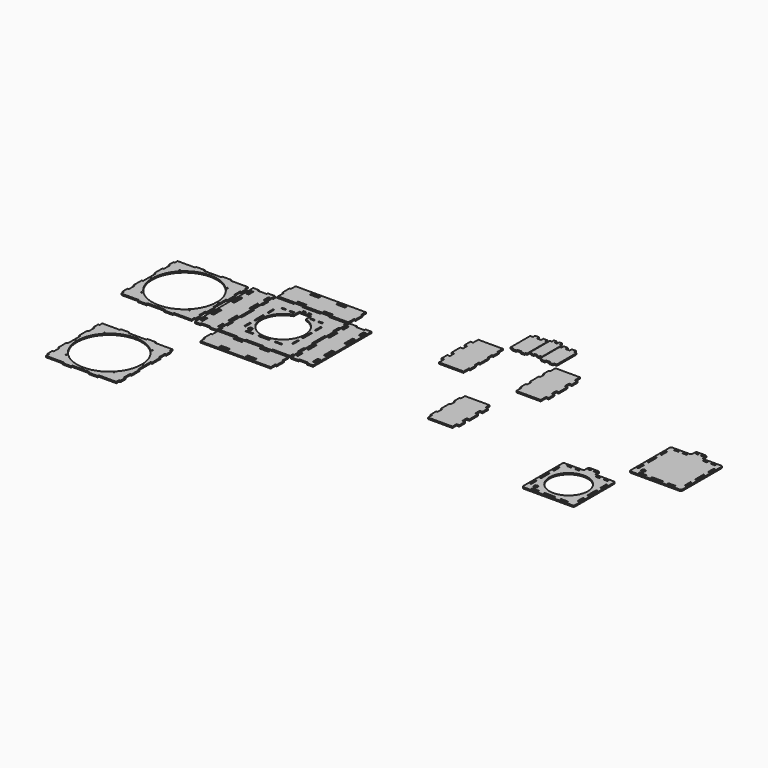
from build123d import *

# Parameters (mm, degrees)
F0_R     = 2
F0_R_2   = 118.6639071569
F1_DEPTH = 5
F0_W     = 32.25
F0_H     = 5
F0_W_2   = 26
F0_R_3   = 7.0999608773
F0_W_3   = 5
F0_H_2   = 26
F0_W_4   = 15
F0_W_5   = 10
F0_H_3   = 22.5386619568
F0_H_4   = 37.4457836151
F0_W_6   = 5.0000161439
F0_W_7   = 40
F0_R_4   = 70


# Not quite as in the source:
# - ends of sketch curves that miss each other by under 0.0002 mm in the source are joined


with BuildPart() as f1:
    # F0 (on Top) → F1 (new body)
    with BuildSketch(Plane.XY):
        Polygon((-1366.6140356064, -884.7837514877), (-1366.6140356064, -897.4375081062), (-1302.1140356064, -897.4375081062), (-1302.1140356064, -902.4375081062), (-1269.8640356064, -902.4375081062), (-1269.8640356064, -897.4375081062), (-1205.3640356064, -897.4375081062), (-1205.3640356064, -902.4375081062), (-1173.1140356064, -902.4375081062), (-1173.1140356064, -897.4375081062), (-1108.6140356064, -897.4375081062), (-1108.6140356064, -884.7837514877), (-1103.6140356064, -884.7837514877), (-1103.6140356064, -862.2450895309), (-1108.6140356064, -862.2450895309), (-1108.6140356064, -834.8589010239), (-1103.6140356064, -834.8589010239), (-1103.6140356064, -797.4131174088), (-1108.6140356064, -797.4131174088), (-1108.6140356064, -739.4618988037), (-1103.6140356064, -739.4618988037), (-1103.6140356064, -702.0161151886), (-1108.6140356064, -702.0161151886), (-1108.6140356064, -674.6299266815), (-1103.6140356064, -674.6299266815), (-1103.6140356064, -652.0912647247), (-1108.6140356064, -652.0912647247), (-1108.6140356064, -639.4375081062), (-1173.1140356064, -639.4375081062), (-1173.1140356064, -634.4375081062), (-1205.3640356064, -634.4375081062), (-1205.3640356064, -639.4375081062), (-1269.8640356064, -639.4375081062), (-1269.8640356064, -634.4375081062), (-1302.1140356064, -634.4375081062), (-1302.1140356064, -639.4375081062), (-1366.6140356064, -639.4375081062), (-1366.6140356064, -652.0912647247), (-1371.6140356064, -652.0912647247), (-1371.6140356064, -674.6299266815), (-1366.6140356064, -674.6299266815), (-1366.6140356064, -702.0161151886), (-1371.6140356064, -702.0161151886), (-1371.6140356064, -739.4618988037), (-1366.6140356064, -739.4618988037), (-1366.6140356064, -797.4131174088), (-1371.6140356064, -797.4131174088), (-1371.6140356064, -834.8589010239), (-1366.6140356064, -834.8589010239), (-1366.6140356064, -862.2450895309), (-1371.6140356064, -862.2450895309), (-1371.6140356064, -884.7837514877), align=None)
        with Locations((-1325.1184997782, -855.9419722781)):
            Circle(F0_R, mode=Mode.SUBTRACT)
        with Locations((-1237.6140356064, -892.1875081062)):
            Circle(F0_R, mode=Mode.SUBTRACT)
        with Locations((-1150.1095714345, -855.9419722781)):
            Circle(F0_R, mode=Mode.SUBTRACT)
        with Locations((-1361.3640356064, -768.4375081062)):
            Circle(F0_R, mode=Mode.SUBTRACT)
        with Locations((-1237.6140356064, -768.4375081062)):
            Circle(F0_R_2, mode=Mode.SUBTRACT)
        with Locations((-1113.8640356064, -768.4375081062)):
            Circle(F0_R, mode=Mode.SUBTRACT)
        with Locations((-1325.1184997782, -680.9330439344)):
            Circle(F0_R, mode=Mode.SUBTRACT)
        with Locations((-1150.1095714345, -680.9330439344)):
            Circle(F0_R, mode=Mode.SUBTRACT)
        with BuildLine():
            ThreePointArc((-1237.6140356064, -646.6875081062), (-1239.0282491688, -643.2732945439), (-1235.6140356064, -644.6875081062))
            ThreePointArc((-1235.6140356064, -644.6875081062), (-1236.199822044, -646.1017216686), (-1237.6140356064, -646.6875081062))
        make_face(mode=Mode.SUBTRACT)
    extrude(amount=F1_DEPTH)


with BuildPart() as f1b:
    # F0 (on Top) → F1, piece 2 (new body)
    with BuildSketch(Plane.XY):
        Polygon((-1293.2458279068, -1321.7081812524), (-1293.2458279068, -1334.3619378709), (-1228.7458279068, -1334.3619378709), (-1228.7458279068, -1339.3619378709), (-1196.4958279068, -1339.3619378709), (-1196.4958279068, -1334.3619378709), (-1131.9958279068, -1334.3619378709), (-1131.9958279068, -1339.3619378709), (-1099.7458279068, -1339.3619378709), (-1099.7458279068, -1334.3619378709), (-1035.2458279068, -1334.3619378709), (-1035.2458279068, -1321.7081812524), (-1030.2458279068, -1321.7081812524), (-1030.2458279068, -1299.1695192956), (-1035.2458279068, -1299.1695192956), (-1035.2458279068, -1271.7833307885), (-1030.2458279068, -1271.7833307885), (-1030.2458279068, -1234.3375471734), (-1035.2458279068, -1234.3375471734), (-1035.2458279068, -1176.3863285683), (-1030.2458279068, -1176.3863285683), (-1030.2458279068, -1138.9405449532), (-1035.2458279068, -1138.9405449532), (-1035.2458279068, -1111.5543564461), (-1030.2458279068, -1111.5543564461), (-1030.2458279068, -1089.0156944894), (-1035.2458279068, -1089.0156944894), (-1035.2458279068, -1076.3619378709), (-1099.7458279068, -1076.3619378709), (-1099.7458279068, -1071.3619378709), (-1131.9958279068, -1071.3619378709), (-1131.9958279068, -1076.3619378709), (-1196.4958279068, -1076.3619378709), (-1196.4958279068, -1071.3619378709), (-1228.7458279068, -1071.3619378709), (-1228.7458279068, -1076.3619378709), (-1293.2458279068, -1076.3619378709), (-1293.2458279068, -1089.0156944894), (-1298.2458279068, -1089.0156944894), (-1298.2458279068, -1111.5543564461), (-1293.2458279068, -1111.5543564461), (-1293.2458279068, -1138.9405449532), (-1298.2458279068, -1138.9405449532), (-1298.2458279068, -1176.3863285683), (-1293.2458279068, -1176.3863285683), (-1293.2458279068, -1234.3375471734), (-1298.2458279068, -1234.3375471734), (-1298.2458279068, -1271.7833307885), (-1293.2458279068, -1271.7833307885), (-1293.2458279068, -1299.1695192956), (-1298.2458279068, -1299.1695192956), (-1298.2458279068, -1321.7081812524), align=None)
        with Locations((-1251.7502920787, -1292.8664020427)):
            Circle(F0_R, mode=Mode.SUBTRACT)
        with Locations((-1164.2458279068, -1329.1119378709)):
            Circle(F0_R, mode=Mode.SUBTRACT)
        with Locations((-1287.9958279068, -1205.3619378709)):
            Circle(F0_R, mode=Mode.SUBTRACT)
        with Locations((-1164.2458279068, -1205.3619378709)):
            Circle(F0_R_2, mode=Mode.SUBTRACT)
        with Locations((-1076.741363735, -1292.8664020427)):
            Circle(F0_R, mode=Mode.SUBTRACT)
        with Locations((-1040.4958279068, -1205.3619378709)):
            Circle(F0_R, mode=Mode.SUBTRACT)
        with Locations((-1251.7502920787, -1117.857473699)):
            Circle(F0_R, mode=Mode.SUBTRACT)
        with BuildLine():
            ThreePointArc((-1164.2458279068, -1083.6119378709), (-1165.6600414692, -1080.1977243085), (-1162.2458279068, -1081.6119378709))
            ThreePointArc((-1162.2458279068, -1081.6119378709), (-1162.8316143445, -1083.0261514332), (-1164.2458279068, -1083.6119378709))
        make_face(mode=Mode.SUBTRACT)
        with Locations((-1076.741363735, -1117.857473699)):
            Circle(F0_R, mode=Mode.SUBTRACT)
    extrude(amount=F1_DEPTH)


with BuildPart() as f1c:
    # F0 (on Top) → F1, piece 3 (new body)
    with BuildSketch(Plane.XY):
        Polygon((-1004.6137704086, -965.3843326569), (-1004.6137704086, -971.6343326569), (-1004.6137704086, -981.6343326569), (-1004.6137704086, -986.6343326569), (-746.6137704086, -986.6343326569), (-746.6137704086, -981.6343326569), (-746.6137704086, -965.3843326569), (-741.6137704086, -965.3843326569), (-741.6137704086, -932.8843326569), (-746.6137704086, -932.8843326569), (-746.6137704086, -911.6343326569), (-746.6137704086, -906.6343326569), (-1004.6137704086, -906.6343326569), (-1004.6137704086, -911.6343326569), (-1004.6137704086, -932.8843326569), (-1009.6137704086, -932.8843326569), (-1009.6137704086, -965.3843326569), align=None)
        Polygon((-907.8637704086, -971.6343326569), (-907.8637704086, -976.6343326569), (-907.8637704086, -981.6343326569), (-940.1137704086, -981.6343326569), (-940.1137704086, -976.6343326569), (-940.1137704086, -971.6343326569), align=None, mode=Mode.SUBTRACT)
        with Locations((-923.9887704086, -914.1343326569)):
            Rectangle(F0_W, F0_H, mode=Mode.SUBTRACT)
        Polygon((-811.1137704086, -971.6343326569), (-811.1137704086, -976.6343326569), (-811.1137704086, -981.6343326569), (-843.3637704086, -981.6343326569), (-843.3637704086, -976.6343326569), (-843.3637704086, -971.6343326569), align=None, mode=Mode.SUBTRACT)
        with Locations((-827.2387704086, -914.1343326569)):
            Rectangle(F0_W, F0_H, mode=Mode.SUBTRACT)
    extrude(amount=F1_DEPTH)


with BuildPart() as f1d:
    # F0 (on Top) → F1, piece 4 (new body)
    with BuildSketch(Plane.XY):
        Polygon((-907.8637704086, -634.4375081062), (-940.1137704086, -634.4375081062), (-940.1137704086, -639.4375081062), (-1004.6137704086, -639.4375081062), (-1004.6137704086, -652.0912647247), (-1009.6137704086, -652.0912647247), (-1009.6137704086, -674.6299266815), (-1004.6137704086, -674.6299266815), (-1004.6137704086, -678.4375081062), (-1004.6137704086, -702.0161151886), (-1009.6137704086, -702.0161151886), (-1009.6137704086, -718.4375081062), (-1009.6137704086, -739.4618988037), (-1004.6137704086, -739.4618988037), (-1004.6137704086, -748.4375081062), (-1004.6137704086, -788.3375081062), (-1004.6137704086, -788.4375081062), (-1004.6137704086, -797.4131174088), (-1009.6137704086, -797.4131174088), (-1009.6137704086, -818.4375081062), (-1009.6137704086, -834.8589010239), (-1004.6137704086, -834.8589010239), (-1004.6137704086, -858.4375081062), (-1004.6137704086, -862.2450895309), (-1009.6137704086, -862.2450895309), (-1009.6137704086, -884.7837514877), (-1004.6137704086, -884.7837514877), (-1004.6137704086, -897.4375081062), (-940.1137704086, -897.4375081062), (-940.1137704086, -902.4375081062), (-907.8637704086, -902.4375081062), (-907.8637704086, -897.4375081062), (-843.3637704086, -897.4375081062), (-843.3637704086, -902.4375081062), (-811.1137704086, -902.4375081062), (-811.1137704086, -897.4375081062), (-746.6137704086, -897.4375081062), (-746.6137704086, -884.7837514877), (-741.6137704086, -884.7837514877), (-741.6137704086, -862.2450895309), (-746.6137704086, -862.2450895309), (-746.6137704086, -858.4375081062), (-746.6137704086, -834.8589010239), (-741.6137704086, -834.8589010239), (-741.6137704086, -818.4375081062), (-741.6137704086, -797.4131174088), (-746.6137704086, -797.4131174088), (-746.6137704086, -788.3375081062), (-746.6137704086, -748.4375081062), (-746.6137704086, -739.4618988037), (-741.6137704086, -739.4618988037), (-741.6137704086, -718.4375081062), (-741.6137704086, -702.0161151886), (-746.6137704086, -702.0161151886), (-746.6137704086, -678.4375081062), (-746.6137704086, -674.6299266815), (-741.6137704086, -674.6299266815), (-741.6137704086, -652.0912647247), (-746.6137704086, -652.0912647247), (-746.6137704086, -639.4375081062), (-811.1137704086, -639.4375081062), (-811.1137704086, -634.4375081062), (-843.3637704086, -634.4375081062), (-843.3637704086, -639.4375081062), (-907.8637704086, -639.4375081062), align=None)
        with Locations((-928.6137704086, -855.9375081062)):
            Rectangle(F0_W_2, F0_H, mode=Mode.SUBTRACT)
        Polygon((-895.6137704086, -858.4375081062), (-895.6137704086, -853.4375081062), (-855.6137704086, -853.4375081062), (-855.6137704086, -858.4375081062), (-875.6137704086, -858.4375081062), align=None, mode=Mode.SUBTRACT)
        with Locations((-940.6262636185, -837.5561237335)):
            Circle(F0_R_3, mode=Mode.SUBTRACT)
        with Locations((-963.1137704086, -821.4375081062)):
            Rectangle(F0_W_3, F0_H_2, mode=Mode.SUBTRACT)
        Polygon((-960.6137704086, -748.4375081062), (-960.6137704086, -768.4375081062), (-960.6137704086, -788.4375081062), (-965.6137704086, -788.4375081062), (-965.6137704086, -748.4375081062), align=None, mode=Mode.SUBTRACT)
        with BuildLine():
            ThreePointArc((-955.6137704086, -768.4375081062), (-939.4886480993, -720.2711297911), (-897.6137704086, -691.5219700141))
            Line((-897.6137704086, -691.5219700141), (-897.6137704086, -666.4375081062))
            Line((-897.6137704086, -666.4375081062), (-875.6137704086, -666.4375081062))
            Line((-875.6137704086, -666.4375081062), (-870.7256383133, -666.4375081062))
            Line((-870.7256383133, -666.4375081062), (-853.6137704086, -666.4375081062))
            Line((-853.6137704086, -666.4375081062), (-853.6137704086, -691.5219700141))
            ThreePointArc((-853.6137704086, -691.5219700141), (-811.7388927179, -720.2711297911), (-795.6137704086, -768.4375081062))
            ThreePointArc((-795.6137704086, -768.4375081062), (-819.0452279137, -825.0060506012), (-875.6137704086, -848.4375081062))
            ThreePointArc((-875.6137704086, -848.4375081062), (-932.1823129036, -825.0060506012), (-955.6137704086, -768.4375081062))
        make_face(mode=Mode.SUBTRACT)
        with Locations((-963.1137704086, -715.4375081062)):
            Rectangle(F0_W_3, F0_H_2, mode=Mode.SUBTRACT)
        with Locations((-822.6137704086, -855.9375081062)):
            Rectangle(F0_W_2, F0_H, mode=Mode.SUBTRACT)
        with Locations((-788.1137704086, -821.4375081062)):
            Rectangle(F0_W_3, F0_H_2, mode=Mode.SUBTRACT)
        Polygon((-790.6137704086, -768.4375081062), (-790.6137704086, -748.4375081062), (-785.6137704086, -748.4375081062), (-785.6137704086, -768.4375081062), (-785.6137704086, -788.4375081062), (-790.6137704086, -788.4375081062), align=None, mode=Mode.SUBTRACT)
        with Locations((-788.1137704086, -715.4375081062)):
            Rectangle(F0_W_3, F0_H_2, mode=Mode.SUBTRACT)
        with Locations((-943.1137704086, -680.9375081062)):
            Rectangle(F0_W_4, F0_H, mode=Mode.SUBTRACT)
        with Locations((-913.1137704086, -680.9375081062)):
            Rectangle(F0_W_4, F0_H, mode=Mode.SUBTRACT)
        with Locations((-885.6137704086, -658.9375081062)):
            Rectangle(F0_W_5, F0_H, mode=Mode.SUBTRACT)
        with Locations((-838.1137704086, -680.9375081062)):
            Rectangle(F0_W_4, F0_H, mode=Mode.SUBTRACT)
        with Locations((-808.1137704086, -680.9375081062)):
            Rectangle(F0_W_4, F0_H, mode=Mode.SUBTRACT)
        with Locations((-865.6137704086, -658.9375081062)):
            Rectangle(F0_W_5, F0_H, mode=Mode.SUBTRACT)
    extrude(amount=F1_DEPTH)


with BuildPart() as f1e:
    # F0 (on Top) → F1, piece 5 (new body)
    with BuildSketch(Plane.XY):
        Polygon((-679.8637704086, -634.4375081062), (-679.8637704086, -639.5375081062), (-696.1137704086, -639.5375081062), (-712.3637704086, -639.5375081062), (-712.3637704086, -634.4375081062), (-728.6137704086, -634.4375081062), (-733.6137704086, -634.4375081062), (-738.6137704086, -634.4375081062), (-738.6137704086, -678.4375081062), (-738.6137704086, -858.4375081062), (-738.6137704086, -902.4375081062), (-733.6137704086, -902.4375081062), (-728.6137704086, -902.4375081062), (-712.3637704086, -902.4375081062), (-712.3637704086, -897.4375081062), (-679.8637704086, -897.4375081062), (-679.8637704086, -902.4375081062), (-663.6137704086, -902.4375081062), (-658.6137704086, -902.4375081062), (-658.6137704086, -634.4375081062), (-663.6137704086, -634.4375081062), align=None)
        with Locations((-731.1137704086, -873.5144205093)):
            Rectangle(F0_W_3, F0_H_3, mode=Mode.SUBTRACT)
        Polygon((-673.6137704086, -862.2450895309), (-668.6137704086, -862.2450895309), (-663.6137704086, -862.2450895309), (-663.6137704086, -884.7837514877), (-668.6137704086, -884.7837514877), (-673.6137704086, -884.7837514877), align=None, mode=Mode.SUBTRACT)
        with Locations((-731.1137704086, -816.1360092163)):
            Rectangle(F0_W_3, F0_H_4, mode=Mode.SUBTRACT)
        Polygon((-673.6137704086, -797.4131174088), (-668.6137704086, -797.4131174088), (-663.6137704086, -797.4131174088), (-663.6137704086, -834.8589010239), (-668.6137704086, -834.8589010239), (-673.6137704086, -834.8589010239), align=None, mode=Mode.SUBTRACT)
        Polygon((-733.6137704086, -702.0161151886), (-728.6137704086, -702.0161151886), (-728.6137704086, -739.4618988037), (-733.6137704086, -739.4618988037), (-733.6137704086, -718.4375081062), align=None, mode=Mode.SUBTRACT)
        Polygon((-668.6137704086, -739.4618988037), (-673.6137704086, -739.4618988037), (-673.6137704086, -702.0161151886), (-668.6137704086, -702.0161151886), (-663.6137704086, -702.0161151886), (-663.6137704086, -739.4618988037), align=None, mode=Mode.SUBTRACT)
        with Locations((-731.1137704086, -663.3605957031)):
            Rectangle(F0_W_3, F0_H_3, mode=Mode.SUBTRACT)
        Polygon((-673.6137704086, -652.0912647247), (-668.6137704086, -652.0912647247), (-663.6137704086, -652.0912647247), (-663.6137704086, -674.6299266815), (-668.6137704086, -674.6299266815), (-673.6137704086, -674.6299266815), align=None, mode=Mode.SUBTRACT)
    extrude(amount=F1_DEPTH)


with BuildPart() as f1f:
    # F0 (on Top) → F1, piece 6 (new body)
    with BuildSketch(Plane.XY):
        Polygon((-1017.6137704086, -634.4375081062), (-1022.6137704086, -634.4375081062), (-1038.8637704086, -634.4375081062), (-1038.8637704086, -639.5375081062), (-1055.1137704086, -639.5375081062), (-1071.3637704086, -639.5375081062), (-1071.3637704086, -634.4375081062), (-1087.6137704086, -634.4375081062), (-1092.6137704086, -634.4375081062), (-1092.6137704086, -902.4375081062), (-1087.6137704086, -902.4375081062), (-1071.3637704086, -902.4375081062), (-1071.3637704086, -897.4375081062), (-1038.8637704086, -897.4375081062), (-1038.8637704086, -902.4375081062), (-1022.6137704086, -902.4375081062), (-1017.6137704086, -902.4375081062), (-1012.6137704086, -902.4375081062), (-1012.6137704086, -858.4375081062), (-1012.6137704086, -678.4375081062), (-1012.6137704086, -634.4375081062), align=None)
        Polygon((-1082.6137704086, -884.7837514877), (-1087.6137704086, -884.7837514877), (-1087.6137704086, -862.2450895309), (-1082.6137704086, -862.2450895309), (-1077.6137704086, -862.2450895309), (-1077.6137704086, -884.7837514877), align=None, mode=Mode.SUBTRACT)
        with Locations((-1020.1137704086, -873.5144205093)):
            Rectangle(F0_W_3, F0_H_3, mode=Mode.SUBTRACT)
        Polygon((-1082.6137704086, -834.8589010239), (-1087.6137704086, -834.8589010239), (-1087.6137704086, -797.4131174088), (-1082.6137704086, -797.4131174088), (-1077.6137704086, -797.4131174088), (-1077.6137704086, -834.8589010239), align=None, mode=Mode.SUBTRACT)
        with Locations((-1020.1137704086, -816.1360092163)):
            Rectangle(F0_W_3, F0_H_4, mode=Mode.SUBTRACT)
        Polygon((-1087.6137704086, -739.4618988037), (-1087.6137704086, -702.0161151886), (-1082.6137704086, -702.0161151886), (-1077.6137704086, -702.0161151886), (-1077.6137704086, -739.4618988037), (-1082.6137704086, -739.4618988037), align=None, mode=Mode.SUBTRACT)
        Polygon((-1017.6137704086, -739.4618988037), (-1022.6137704086, -739.4618988037), (-1022.6137704086, -702.0161151886), (-1017.6137704086, -702.0161151886), (-1017.6137704086, -718.4375081062), align=None, mode=Mode.SUBTRACT)
        Polygon((-1087.6137704086, -674.6299266815), (-1087.6137704086, -652.0912647247), (-1082.6137704086, -652.0912647247), (-1077.6137704086, -652.0912647247), (-1077.6137704086, -674.6299266815), (-1082.6137704086, -674.6299266815), align=None, mode=Mode.SUBTRACT)
        with Locations((-1020.1137704086, -663.3605957031)):
            Rectangle(F0_W_3, F0_H_3, mode=Mode.SUBTRACT)
    extrude(amount=F1_DEPTH)


with BuildPart() as f1g:
    # F0 (on Top) → F1, piece 7 (new body)
    with BuildSketch(Plane.XY):
        Polygon((-1004.6137704086, -620.2406835556), (-1004.6137704086, -625.2406835556), (-1004.6137704086, -630.2406835556), (-940.1137704086, -630.2406835556), (-746.6137704086, -630.2406835556), (-746.6137704086, -625.2406835556), (-746.6137704086, -603.9906835556), (-741.6137704086, -603.9906835556), (-741.6137704086, -571.4906835556), (-746.6137704086, -571.4906835556), (-746.6137704086, -555.2406835556), (-746.6137704086, -550.2406835556), (-1004.6137704086, -550.2406835556), (-1004.6137704086, -555.2406835556), (-1004.6137704086, -565.2406835556), (-1004.6137704086, -571.4906835556), (-1009.6137704086, -571.4906835556), (-1009.6137704086, -603.9906835556), (-1004.6137704086, -603.9906835556), align=None)
        with Locations((-923.9887704086, -622.7406835556)):
            Rectangle(F0_W, F0_H, mode=Mode.SUBTRACT)
        Polygon((-940.1137704086, -565.2406835556), (-940.1137704086, -560.2406835556), (-940.1137704086, -555.2406835556), (-907.8637704086, -555.2406835556), (-907.8637704086, -560.2406835556), (-907.8637704086, -565.2406835556), align=None, mode=Mode.SUBTRACT)
        with Locations((-827.2387704086, -622.7406835556)):
            Rectangle(F0_W, F0_H, mode=Mode.SUBTRACT)
        Polygon((-811.1137704086, -555.2406835556), (-811.1137704086, -560.2406835556), (-811.1137704086, -565.2406835556), (-843.3637704086, -565.2406835556), (-843.3637704086, -560.2406835556), (-843.3637704086, -555.2406835556), align=None, mode=Mode.SUBTRACT)
    extrude(amount=F1_DEPTH)


with BuildPart() as f1h:
    # F0 (on Top) → F1, piece 8 (new body)
    with BuildSketch(Plane.XY):
        Polygon((-298.4449183991, -662.1296386563), (-298.1309330463, -662.1296386563), (-298.1309330463, -638.1296386563), (-293.1309330463, -638.1296386563), (-293.1309330463, -612.1296386563), (-298.1309330463, -612.1296386563), (-298.1309330463, -592.1296386563), (-293.1309330463, -592.1296386563), (-293.1309330463, -552.1665781096), (-298.1309330463, -552.1665781096), (-298.1309330463, -532.1665781096), (-293.1309330463, -532.1665781096), (-293.1309330463, -506.1665781096), (-298.1309330463, -506.1296386563), (-298.1309330463, -482.1296386563), (-383.1309330463, -482.1296386563), (-388.1309330463, -482.1296386563), (-388.1309330463, -492.7178739505), (-388.1309330463, -506.1296386563), (-398.1309330463, -506.1296386563), (-398.1309330463, -532.1665781096), (-388.1309330463, -532.1665781096), (-388.1309330463, -552.1665781096), (-398.1309330463, -552.1665781096), (-398.1309330463, -592.1296386563), (-388.1309330463, -592.1296386563), (-388.1309330463, -612.1296386563), (-398.1309330463, -612.1296386563), (-398.1309330463, -638.1296386563), (-388.1309330463, -638.1296386563), (-388.1309330463, -651.5783428154), (-388.1309330463, -662.1296386563), align=None)
    extrude(amount=F1_DEPTH)


with BuildPart() as f1i:
    # F0 (on Top) → F1, piece 9 (new body)
    with BuildSketch(Plane.XY):
        Polygon((-286.3878677518, -460.9915268421), (-284.3879467788, -460.9915268421), (-276.3878677518, -460.9915268421), (-276.3878677518, -465.9915268421), (-271.3878677518, -465.9915268421), (-261.3878677518, -465.9915268421), (-261.3878677518, -460.9915268421), (-256.9990215546, -460.9915268421), (-246.3878677518, -460.9915268421), (-246.3878677518, -465.9915268421), (-241.3878677518, -465.9915268421), (-231.3878677518, -465.9915268421), (-231.3878677518, -460.9915268421), (-225.3675460815, -461.0270857811), (-225.3675460815, -371.0271845648), (-231.3878677518, -371.0271845648), (-231.3878677518, -361.0270857811), (-241.3878677518, -361.0270857811), (-246.3878677518, -361.0270857811), (-246.3878677518, -371.0271852235), (-256.4324156498, -371.0271852235), (-261.3878677518, -371.0271852235), (-261.3878677518, -361.0270857811), (-276.3878677518, -361.0270857811), (-276.3878677518, -371.0271852235), (-286.3878677518, -371.0271852235), align=None)
    extrude(amount=F1_DEPTH)


with BuildPart() as f1j:
    # F0 (on Top) → F1, piece 10 (new body)
    with BuildSketch(Plane.XY):
        Polygon((-216.3878677518, -359.7890693303), (-223.3878677518, -359.7890693303), (-223.3878677518, -449.7890693303), (-216.3878677518, -449.7890693303), (-216.3878677518, -454.7890693303), (-206.3878677518, -454.7890693303), (-206.3878677518, -449.7890693303), (-201.4541815716, -449.7890693303), (-201.3215539319, -449.7890693303), (-196.3878677518, -449.7890693303), (-196.3878677518, -454.7890693303), (-186.3878677518, -454.7890693303), (-186.3878677518, -449.7890693303), (-179.3878677518, -449.7890693303), (-179.3878677518, -359.7890693303), (-186.3878677518, -359.7890693303), (-186.3878677518, -354.7890693303), (-186.3878677518, -349.7890693303), (-196.3878677518, -349.7890693303), (-196.3878677518, -354.7890693303), (-196.3878677518, -359.7890693303), (-201.3878677518, -359.7890693303), (-206.3878677518, -359.7890693303), (-206.3878677518, -354.7890693303), (-206.3878677518, -349.7890693303), (-216.3878677518, -349.7890693303), (-216.3878677518, -354.7890693303), align=None)
    extrude(amount=F1_DEPTH)


with BuildPart() as f1k:
    # F0 (on Top) → F1, piece 11 (new body)
    with BuildSketch(Plane.XY):
        Polygon((-177.408189422, -371.0271845648), (-177.408189422, -461.0270857811), (-171.3878677518, -460.9915268421), (-171.3878677518, -465.9915268421), (-161.3878677518, -465.9915268421), (-156.3878677518, -465.9915268421), (-156.3878677518, -460.9915268421), (-145.7767139489, -460.9915268421), (-141.3878677518, -460.9915268421), (-141.3878677518, -465.9915268421), (-131.3878677518, -465.9915268421), (-126.3878677518, -465.9915268421), (-126.3878677518, -460.9915268421), (-118.3877887248, -460.9915268421), (-116.3878677518, -460.9915268421), (-116.3878677518, -371.0271852235), (-126.3878677518, -371.0271852235), (-126.3878677518, -361.0270857811), (-141.3878677518, -361.0270857811), (-141.3878677518, -371.0271852235), (-146.3433198538, -371.0271852235), (-156.3878677518, -371.0271852235), (-156.3878677518, -361.0270857811), (-161.3878677518, -361.0270857811), (-171.3878677518, -361.0270857811), (-171.3878677518, -371.0271845648), align=None)
    extrude(amount=F1_DEPTH)


with BuildPart() as f1l:
    # F0 (on Top) → F1, piece 12 (new body)
    with BuildSketch(Plane.XY):
        Polygon((-104.6448024572, -482.1296386563), (-104.6448024572, -506.1296386563), (-109.6448024572, -506.1665781096), (-109.6448024572, -532.1665781096), (-104.6448024572, -532.1665781096), (-104.6448024572, -552.1665781096), (-109.6448024572, -552.1665781096), (-109.6448024572, -592.1296386563), (-104.6448024572, -592.1296386563), (-104.6448024572, -612.1296386563), (-109.6448024572, -612.1296386563), (-109.6448024572, -638.1296386563), (-104.6448024572, -638.1296386563), (-104.6448024572, -662.1296386563), (-104.3308171044, -662.1296386563), (-14.6448024572, -662.1296386563), (-14.6448024572, -651.5783428154), (-14.6448024572, -638.1296386563), (-4.6448024572, -638.1296386563), (-4.6448024572, -612.1296386563), (-14.6448024572, -612.1296386563), (-14.6448024572, -592.1296386563), (-4.6448024572, -592.1296386563), (-4.6448024572, -552.1665781096), (-14.6448024572, -552.1665781096), (-14.6448024572, -532.1665781096), (-4.6448024572, -532.1665781096), (-4.6448024572, -506.1296386563), (-14.6448024572, -506.1296386563), (-14.6448024572, -492.7178739505), (-14.6448024572, -482.1296386563), (-19.6448024572, -482.1296386563), align=None)
    extrude(amount=F1_DEPTH)


with BuildPart() as f1m:
    # F0 (on Top) → F1, piece 13 (new body)
    with BuildSketch(Plane.XY):
        Polygon((-199.1916574645, -780.1817527555), (-199.1916574645, -798.1817527555), (-204.1916574645, -798.2186922088), (-204.1916574645, -824.2186922088), (-199.1916574645, -824.2186922088), (-199.1916574645, -844.2186922088), (-204.1916574645, -844.2186922088), (-204.1916574645, -884.1817527555), (-199.1916574645, -884.1817527555), (-199.1916574645, -904.1817527555), (-204.1916574645, -904.1817527555), (-204.1916574645, -930.1817527555), (-199.1916574645, -930.1817527555), (-199.1916574645, -948.2556316621), (-199.1916574645, -949.2556316621), (-109.1916574645, -949.2556316621), (-109.1916574645, -938.6673963679), (-109.1916574645, -930.1817527555), (-99.1916574645, -930.1817527555), (-99.1916574645, -904.1817527555), (-109.1916574645, -904.1817527555), (-109.1916574645, -884.1817527555), (-99.1916574645, -884.1817527555), (-99.1916574645, -844.2186922088), (-109.1916574645, -844.2186922088), (-109.1916574645, -824.2186922088), (-99.1916574645, -824.2186922088), (-99.1916574645, -798.1817527555), (-109.1916574645, -798.1817527555), (-109.1916574645, -789.7699880497), (-109.1916574645, -779.1817527555), (-199.1916574645, -779.1817527555), align=None)
    extrude(amount=F1_DEPTH)


with BuildPart() as f1n:
    # F0 (on Top) → F1, piece 14 (new body)
    with BuildSketch(Plane.XY):
        with BuildLine():
            Line((464.3994565253, -847.4577746544), (488.3994726692, -847.4577746544))
            Line((488.3994726692, -847.4577746544), (644.3994565253, -847.4577746544))
            ThreePointArc((644.3994565253, -847.4577746544), (647.9349904312, -845.9933085603), (649.3994565253, -842.4577746544))
            Line((649.3994565253, -842.4577746544), (649.3994565253, -662.4577746544))
            ThreePointArc((649.3994565253, -662.4577746544), (647.9349904312, -658.9222407484), (644.3994565253, -657.4577746544))
            Line((644.3994565253, -657.4577746544), (579.3994565253, -657.4577746544))
            ThreePointArc((579.3994565253, -657.4577746544), (575.8639226194, -655.9933085603), (574.3994565253, -652.4577746544))
            Line((574.3994565253, -652.4577746544), (574.3994565253, -650.476244381))
            Line((574.3994565253, -650.476244381), (574.3994565253, -645.476244381))
            Line((574.3994565253, -645.476244381), (574.3994565253, -640.476244381))
            ThreePointArc((574.3994565253, -640.476244381), (572.9349904312, -636.9406895606), (569.3994565253, -635.4762234665))
            Line((569.3994565253, -635.4762234665), (539.3994565253, -635.4762234665))
            ThreePointArc((539.3994565253, -635.4762234665), (535.8639226194, -636.9406895606), (534.3994565253, -640.4762234665))
            Line((534.3994565253, -640.4762234665), (534.3994565253, -652.4577746544))
            ThreePointArc((534.3994565253, -652.4577746544), (532.9349904312, -655.9933085603), (529.3994565253, -657.4577746544))
            Line((529.3994565253, -657.4577746544), (464.3994565253, -657.4577746544))
            ThreePointArc((464.3994565253, -657.4577746544), (460.8639226194, -658.9222407484), (459.3994565253, -662.4577746544))
            Line((459.3994565253, -662.4577746544), (459.3994565253, -752.4947141076))
            Line((459.3994565253, -752.4947141076), (459.3994565253, -842.4577746544))
            ThreePointArc((459.3994565253, -842.4577746544), (460.8639226194, -845.9933085603), (464.3994565253, -847.4577746544))
        make_face()
        with Locations((501.3994726692, -839.9577746544)):
            Rectangle(F0_W_2, F0_H, mode=Mode.SUBTRACT)
        with Locations((489.3869633155, -821.5763902817)):
            Circle(F0_R_3, mode=Mode.SUBTRACT)
        with Locations((466.8994645973, -805.4577746544)):
            Rectangle(F0_W_6, F0_H_2, mode=Mode.SUBTRACT)
        with Locations((554.3994726692, -839.9577746544)):
            Rectangle(F0_W_7, F0_H, mode=Mode.SUBTRACT)
        with Locations((607.3994726692, -839.9577746544)):
            Rectangle(F0_W_2, F0_H, mode=Mode.SUBTRACT)
        with Locations((641.8994484533, -805.4577746544)):
            Rectangle(F0_W_6, F0_H_2, mode=Mode.SUBTRACT)
        Polygon((469.3994565253, -752.4947141076), (469.3994565253, -772.4577746544), (464.3994565253, -772.4577746544), (464.3994565253, -732.4947141076), (469.3994565253, -732.4947141076), align=None, mode=Mode.SUBTRACT)
        with Locations((466.8994645973, -699.4947141076)):
            Rectangle(F0_W_6, F0_H_2, mode=Mode.SUBTRACT)
        Polygon((639.3994565253, -752.4947141076), (639.3994565253, -732.4947141076), (644.3994565253, -732.4947141076), (644.3994565253, -772.4577746544), (639.3994565253, -772.4577746544), align=None, mode=Mode.SUBTRACT)
        with Locations((641.8994484533, -699.4947141076)):
            Rectangle(F0_W_6, F0_H_2, mode=Mode.SUBTRACT)
        Polygon((479.3994565253, -667.4577746544), (479.3994565253, -662.4577746544), (484.3994565253, -662.4577746544), (494.3994565253, -662.4577746544), (494.3994565253, -667.4577746544), (484.3994565253, -667.4577746544), align=None, mode=Mode.SUBTRACT)
        Polygon((514.3994565253, -667.4577746544), (509.3994565253, -667.4577746544), (509.3994565253, -662.4577746544), (514.3994565253, -662.4577746544), (524.3994565253, -662.4577746544), (524.3994565253, -667.4577746544), align=None, mode=Mode.SUBTRACT)
        Polygon((594.3994565253, -662.4577746544), (599.3994565253, -662.4577746544), (599.3994565253, -667.4577746544), (594.3994565253, -667.4577746544), (584.3994565253, -667.4577746544), (584.3994565253, -662.4577746544), align=None, mode=Mode.SUBTRACT)
        Polygon((629.3994565253, -667.4577746544), (624.3994565253, -667.4577746544), (614.3994565253, -667.4577746544), (614.3994565253, -662.4577746544), (624.3994565253, -662.4577746544), (629.3994565253, -662.4577746544), align=None, mode=Mode.SUBTRACT)
        with Locations((544.3994565253, -642.976244381)):
            Rectangle(F0_W_5, F0_H, mode=Mode.SUBTRACT)
        with Locations((564.3994565253, -642.976244381)):
            Rectangle(F0_W_5, F0_H, mode=Mode.SUBTRACT)
    extrude(amount=F1_DEPTH)


with BuildPart() as f1o:
    # F0 (on Top) → F1, piece 15 (new body)
    with BuildSketch(Plane.XY):
        with BuildLine():
            Line((284.8862236783, -1116.0823865112), (308.8862398223, -1116.0823865112))
            Line((308.8862398223, -1116.0823865112), (464.8862236783, -1116.0823865112))
            ThreePointArc((464.8862236783, -1116.0823865112), (468.4217575843, -1114.6179204171), (469.8862236783, -1111.0823865112))
            Line((469.8862236783, -1111.0823865112), (469.8862236783, -931.0823865112))
            ThreePointArc((469.8862236783, -931.0823865112), (468.4217575843, -927.5468526053), (464.8862236783, -926.0823865112))
            Line((464.8862236783, -926.0823865112), (399.8862236783, -926.0823865112))
            ThreePointArc((399.8862236783, -926.0823865112), (396.3506897724, -924.6179204171), (394.8862236783, -921.0823865112))
            Line((394.8862236783, -921.0823865112), (394.8862236783, -919.1008562378))
            Line((394.8862236783, -919.1008562378), (394.8862236783, -914.1008562378))
            Line((394.8862236783, -914.1008562378), (394.8862236783, -909.1008562378))
            ThreePointArc((394.8862236783, -909.1008562378), (393.4217575843, -905.5653014174), (389.8862236783, -904.1008353233))
            Line((389.8862236783, -904.1008353233), (359.8862236783, -904.1008353233))
            ThreePointArc((359.8862236783, -904.1008353233), (356.3506897724, -905.5653014174), (354.8862236783, -909.1008353233))
            Line((354.8862236783, -909.1008353233), (354.8862236783, -921.0823865112))
            ThreePointArc((354.8862236783, -921.0823865112), (353.4217575843, -924.6179204171), (349.8862236783, -926.0823865112))
            Line((349.8862236783, -926.0823865112), (284.8862236783, -926.0823865112))
            ThreePointArc((284.8862236783, -926.0823865112), (281.3506897724, -927.5468526053), (279.8862236783, -931.0823865112))
            Line((279.8862236783, -931.0823865112), (279.8862236783, -1021.1193259645))
            Line((279.8862236783, -1021.1193259645), (279.8862236783, -1111.0823865112))
            ThreePointArc((279.8862236783, -1111.0823865112), (281.3506897724, -1114.6179204171), (284.8862236783, -1116.0823865112))
        make_face()
        with Locations((321.8862398223, -1108.5823865112)):
            Rectangle(F0_W_2, F0_H, mode=Mode.SUBTRACT)
        with Locations((374.8862398223, -1108.5823865112)):
            Rectangle(F0_W_7, F0_H, mode=Mode.SUBTRACT)
        with Locations((309.8737304685, -1090.2010021385)):
            Circle(F0_R_3, mode=Mode.SUBTRACT)
        with Locations((287.3862317503, -1074.0823865112)):
            Rectangle(F0_W_6, F0_H_2, mode=Mode.SUBTRACT)
        Polygon((289.8862236783, -1021.1193259645), (289.8862236783, -1041.0823865112), (284.8862236783, -1041.0823865112), (284.8862236783, -1001.1193259645), (289.8862236783, -1001.1193259645), align=None, mode=Mode.SUBTRACT)
        with Locations((374.8862236783, -1021.1008562378)):
            Circle(F0_R_4, mode=Mode.SUBTRACT)
        with Locations((427.8862398223, -1108.5823865112)):
            Rectangle(F0_W_2, F0_H, mode=Mode.SUBTRACT)
        with Locations((462.3862156064, -1074.0823865112)):
            Rectangle(F0_W_6, F0_H_2, mode=Mode.SUBTRACT)
        Polygon((459.8862236783, -1021.1193259645), (459.8862236783, -1001.1193259645), (464.8862236783, -1001.1193259645), (464.8862236783, -1041.0823865112), (459.8862236783, -1041.0823865112), align=None, mode=Mode.SUBTRACT)
        with Locations((287.3862317503, -968.1193259645)):
            Rectangle(F0_W_6, F0_H_2, mode=Mode.SUBTRACT)
        Polygon((299.8862236783, -936.0823865112), (299.8862236783, -931.0823865112), (304.8862236783, -931.0823865112), (314.8862236783, -931.0823865112), (314.8862236783, -936.0823865112), (304.8862236783, -936.0823865112), align=None, mode=Mode.SUBTRACT)
        Polygon((334.8862236783, -936.0823865112), (329.8862236783, -936.0823865112), (329.8862236783, -931.0823865112), (334.8862236783, -931.0823865112), (344.8862236783, -931.0823865112), (344.8862236783, -936.0823865112), align=None, mode=Mode.SUBTRACT)
        with Locations((364.8862236783, -911.6008562378)):
            Rectangle(F0_W_5, F0_H, mode=Mode.SUBTRACT)
        with Locations((384.8862236783, -911.6008562378)):
            Rectangle(F0_W_5, F0_H, mode=Mode.SUBTRACT)
        Polygon((414.8862236783, -931.0823865112), (419.8862236783, -931.0823865112), (419.8862236783, -936.0823865112), (414.8862236783, -936.0823865112), (404.8862236783, -936.0823865112), (404.8862236783, -931.0823865112), align=None, mode=Mode.SUBTRACT)
        Polygon((449.8862236783, -936.0823865112), (444.8862236783, -936.0823865112), (434.8862236783, -936.0823865112), (434.8862236783, -931.0823865112), (444.8862236783, -931.0823865112), (449.8862236783, -931.0823865112), align=None, mode=Mode.SUBTRACT)
        with Locations((462.3862156064, -968.1193259645)):
            Rectangle(F0_W_6, F0_H_2, mode=Mode.SUBTRACT)
    extrude(amount=F1_DEPTH)


solid = Compound([f1.part, f1b.part, f1c.part, f1d.part, f1e.part, f1f.part, f1g.part, f1h.part, f1i.part, f1j.part, f1k.part, f1l.part, f1m.part, f1n.part, f1o.part])
